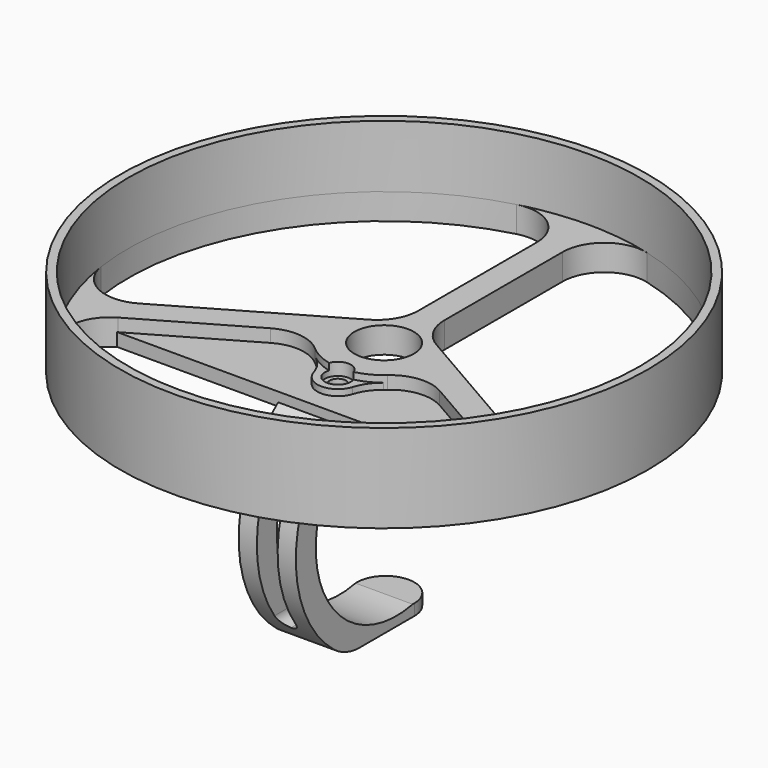
from build123d import *

# Parameters (mm, degrees)
F0_R         = 32.258
F0_R_2       = 3.6322
F1_DEPTH     = 3.175
F4_DEPTH     = 3.4925
F5_W         = 2.54
F5_H         = 20.32
F6_DEPTH     = 25.4
F7_R         = 1.26999
F8_R         = 3.4798
F9_R         = 32.258
F9_R_2       = 31.242
F10_DEPTH    = 7.62
F12_DEPTH    = 1.5748
F13_T1_DEPTH = 3.175
F13_T3_DEPTH = 1.5748
F14_R        = 2.5029708097
F15_DEPTH    = 0.762
F16_T1_DEPTH = 0.762
F17_R        = 1.016
F18_DEPTH    = 25.4
F19_R        = 1.5875
F20_DEPTH    = 1.524


# Not quite as in the source:
# - a fillet or chamfer that OpenCascade refuses, or shapes differently, is made with other operations: its cross-section is extruded or revolved along the edge and cut away or added
# - a fillet or chamfer is up to 0.001 mm smaller than in the source, because OpenCascade refuses the exact size


with BuildPart() as f1:
    # F0 (on Top) → F1 (new body)
    with BuildSketch(Plane.XY):
        Circle(F0_R)
        with BuildLine():
            ThreePointArc((27.6984583499, -14.4519192165), (0, -31.242), (-27.6984583499, -14.4519192165))
            Line((-27.6984583499, -14.4519192165), (-23.1550479516, -11.82878))
            Line((-23.1550479516, -11.82878), (23.1550479516, -11.82878))
            Line((23.1550479516, -11.82878), (27.6984583499, -14.4519192165))
        make_face(mode=Mode.SUBTRACT)
        with BuildLine():
            ThreePointArc((-1.5875, 4.2197649224), (-1.9273330318, 4.0757771817), (-2.25425, 3.904475533))
            Line((-2.25425, 3.904475533), (-29.0274080844, -11.5530144941))
            ThreePointArc((-29.0274080844, -11.5530144941), (-26.2927422142, 16.8746635777), (-1.5875, 31.2016411067))
            Line((-1.5875, 31.2016411067), (-1.5875, 4.2197649224))
        make_face(mode=Mode.SUBTRACT)
        Circle(F0_R_2, mode=Mode.SUBTRACT)
        with BuildLine():
            Line((29.0274080844, -11.5530144941), (2.25425, 3.904475533))
            ThreePointArc((2.25425, 3.904475533), (1.9273330318, 4.0757771817), (1.5875, 4.2197649224))
            Line((1.5875, 4.2197649224), (1.5875, 31.2016411067))
            ThreePointArc((1.5875, 31.2016411067), (26.2927422142, 16.8746635777), (29.0274080844, -11.5530144941))
        make_face(mode=Mode.SUBTRACT)
    extrude(amount=-F1_DEPTH)

    # F3 (on offset) → F4 (join, symmetric)
    with BuildSketch(Plane.YZ):
        with BuildLine():
            ThreePointArc((0, -26.9952715967), (-14.4117945702, -18.019693004), (-6.1718963048, -3.175))
            Line((-6.1718963048, -3.175), (-6.1718963048, -2.7284894604))
            Line((-6.1718963048, -2.7284894604), (-11.8285217471, -2.7284894604))
            ThreePointArc((-11.8285217471, -2.7284894604), (-17.8532575218, -14.8291637745), (-11.9875892757, -27.0077390621))
            ThreePointArc((-11.9875892757, -27.0077390621), (-10.1388723772, -28.0174760831), (-8.0615554064, -28.3668715967))
            Line((-8.0615554064, -28.3668715967), (3.7295622751, -28.3668715967))
            Line((3.7295622751, -28.3668715967), (3.7295622751, -26.9952715967))
            Line((3.7295622751, -26.9952715967), (0, -26.9952715967))
        make_face()
    extrude(amount=F4_DEPTH, both=True)

    # F5 (on Front) → F6 (cut)
    with BuildSketch(Plane.XZ):
        with Locations((0, -14.732)):
            Rectangle(F5_W, F5_H)
    extrude(amount=F6_DEPTH, mode=Mode.SUBTRACT)

    # F7 (radius 1.27 in the source; OpenCascade refuses exactly that, so slightly less here)
    f7_edges = [f1.edges().sort_by_distance(p)[0] for p in [
        (1.27, -11.496811, -4.572),
        (-1.27, -11.496811, -4.572),
        (1.27, -11.960099, -24.892),
        (-1.27, -11.960099, -24.892),
    ]]
    fillet(f7_edges, radius=F7_R)

    # F8
    f8_edges = [f1.edges().sort_by_distance(p)[0] for p in [
        (-3.4925, 3.729562, -27.681072),
        (3.4925, 3.729562, -27.681072),
    ]]
    fillet(f8_edges, radius=F8_R)

    # F9 (on face) → F10 (join)
    with BuildSketch(Plane.XY):
        Circle(F9_R)
        Circle(F9_R_2, mode=Mode.SUBTRACT)
    extrude(amount=F10_DEPTH)

    # F11 (on face) → F12 (cut)
    with BuildSketch(Plane.XY):
        with BuildLine():
            Line((-6.35, -2.1263810414), (-23.1550479516, -11.82878))
            Line((-23.1550479516, -11.82878), (-23.1550479516, -13.7292239815))
            Line((-23.1550479516, -13.7292239815), (23.1550479516, -13.8936461881))
            Line((23.1550479516, -13.8936461881), (23.1550479516, -11.82878))
            Line((23.1550479516, -11.82878), (6.35, -2.1263810414))
            ThreePointArc((6.35, -2.1263810414), (0, -6.6965660105), (-6.35, -2.1263810414))
        make_face()
    extrude(amount=-F12_DEPTH, mode=Mode.SUBTRACT)

    # F13: fillet of radius 5.08 on 10 edges, made by hand

    # F13_s2 → F13_t1 (join)
    with BuildSketch(Plane.XY.offset(-3.175)):
        with BuildLine():
            ThreePointArc((1.5875, 7.2223631924), (2.2680909488, 4.6823631924), (4.1275, 2.8229541412))
            Line((4.1275, 2.8229541412), (3.8735, 2.3830132361))
            ThreePointArc((3.8735, 2.3830132361), (2.00025, 3.4645346278), (1.4086267606, 3.7442984522))
            Line((1.4086267606, 3.7442984522), (1.0795, 4.2197649224))
            Line((1.0795, 4.2197649224), (1.0795, 7.2223631924))
            Line((1.0795, 7.2223631924), (1.5875, 7.2223631924))
        make_face()
        with BuildLine():
            ThreePointArc((-4.1275, 2.8229541412), (-2.2680909488, 4.6823631924), (-1.5875, 7.2223631924))
            Line((-1.5875, 7.2223631924), (-1.0795, 7.2223631924))
            Line((-1.0795, 7.2223631924), (-1.0795, 4.2197649224))
            Line((-1.0795, 4.2197649224), (-1.4086267606, 3.7442984522))
            ThreePointArc((-1.4086267606, 3.7442984522), (-2.00025, 3.4645346278), (-3.8735, 2.3830132361))
            Line((-3.8735, 2.3830132361), (-4.1275, 2.8229541412))
        make_face()
        with BuildLine():
            ThreePointArc((1.5875, 25.2981162886), (3.5667318521, 29.3219995987), (7.9621601942, 30.2103718786))
            ThreePointArc((7.9621601942, 30.2103718786), (4.8004849887, 30.870988126), (1.5875, 31.2016411067))
            Line((1.5875, 31.2016411067), (1.5875, 25.2981162886))
        make_face()
        with BuildLine():
            ThreePointArc((-7.9621601942, 30.2103718786), (-3.5667318521, 29.3219995987), (-1.5875, 25.2981162886))
            Line((-1.5875, 25.2981162886), (-1.5875, 31.2016411067))
            ThreePointArc((-1.5875, 31.2016411067), (-4.8004849887, 30.870988126), (-7.9621601942, 30.2103718786))
        make_face()
        with BuildLine():
            ThreePointArc((-23.0901860951, -11.7913319897), (-25.5388151591, -15.2315851298), (-24.5405134922, -19.3345742528))
            ThreePointArc((-24.5405134922, -19.3345742528), (-26.2333304182, -16.9668777083), (-27.6984583499, -14.4519192165))
            Line((-27.6984583499, -14.4519192165), (-23.0901860951, -11.7913319897))
        make_face()
        with BuildLine():
            ThreePointArc((-23.3346480943, -8.2662979814), (-28.0816389218, -8.4424316835), (-30.8988516077, -4.6177411496))
            ThreePointArc((-30.8988516077, -4.6177411496), (-30.1631174493, -8.1393433235), (-29.0274080844, -11.5530144941))
            Line((-29.0274080844, -11.5530144941), (-23.3346480943, -8.2662979814))
        make_face()
        with BuildLine():
            ThreePointArc((24.5405134922, -19.3345742528), (25.5388151591, -15.2315851298), (23.0901860951, -11.7913319897))
            Line((23.0901860951, -11.7913319897), (27.6984583499, -14.4519192165))
            ThreePointArc((27.6984583499, -14.4519192165), (26.2333304182, -16.9668777083), (24.5405134922, -19.3345742528))
        make_face()
        with BuildLine():
            ThreePointArc((30.8988516077, -4.6177411496), (28.0816389218, -8.4424316835), (23.3346480943, -8.2662979814))
            Line((23.3346480943, -8.2662979814), (29.0274080844, -11.5530144941))
            ThreePointArc((29.0274080844, -11.5530144941), (30.1631174493, -8.1393433235), (30.8988516077, -4.6177411496))
        make_face()
    extrude(amount=F13_T1_DEPTH)

    # F13_s4 → F13_t3 (join)
    with BuildSketch(Plane.XY.offset(-1.5748)):
        with BuildLine():
            ThreePointArc((4.4329020877, -5.0193002913), (7.2889409664, -3.7722686868), (10.3356916982, -4.4275212163))
            Line((10.3356916982, -4.4275212163), (6.35, -2.1263810414))
            ThreePointArc((6.35, -2.1263810414), (5.5821133816, -3.6991899827), (4.4329020877, -5.0193002913))
        make_face()
        with BuildLine():
            ThreePointArc((-10.3356916982, -4.4275212163), (-7.2889409664, -3.7722686868), (-4.4329020877, -5.0193002913))
            ThreePointArc((-4.4329020877, -5.0193002913), (-5.5821133816, -3.6991899827), (-6.35, -2.1263810414))
            Line((-6.35, -2.1263810414), (-10.3356916982, -4.4275212163))
        make_face()
    extrude(amount=F13_T3_DEPTH)

    # F14 (on face) → F15 (join)
    with BuildSketch(Plane.XY.offset(-1.5748)):
        with Locations((0, -7.0612)):
            Circle(F14_R)
    extrude(amount=F15_DEPTH)

    # F16: fillet of radius 5.08 on 2 edges, made by hand

    # F16_s2 → F16_t1 (join)
    with BuildSketch(Plane.XY.offset(-1.5748)):
        with BuildLine():
            ThreePointArc((-4.123339334, -5.2765584494), (-3.0648098759, -6.4018902356), (-2.3934920763, -7.7933601976))
            ThreePointArc((-2.3934920763, -7.7933601976), (-2.5027259003, -7.02618654), (-2.3720733098, -6.2623689245))
            ThreePointArc((-2.3720733098, -6.2623689245), (-3.2848975519, -5.8355329154), (-4.123339334, -5.2765584494))
        make_face()
        with BuildLine():
            ThreePointArc((4.123339334, -5.2765584494), (3.0648098759, -6.4018902356), (2.3934920763, -7.7933601976))
            ThreePointArc((2.3934920763, -7.7933601976), (2.5027259003, -7.02618654), (2.3720733098, -6.2623689245))
            ThreePointArc((2.3720733098, -6.2623689245), (3.2848975519, -5.8355329154), (4.123339334, -5.2765584494))
        make_face()
    extrude(amount=F16_T1_DEPTH)

    # F17 (on face) → F18 (cut)
    with BuildSketch(Plane.XY):
        with Locations((0, -7.0612)):
            Circle(F17_R)
    extrude(amount=-F18_DEPTH, mode=Mode.SUBTRACT)

    # F19 (on face) → F20 (cut)
    with BuildSketch(Plane.XY):
        with Locations((0, -7.0612)):
            Circle(F19_R)
    extrude(amount=-F20_DEPTH, mode=Mode.SUBTRACT)


solid = f1.part
